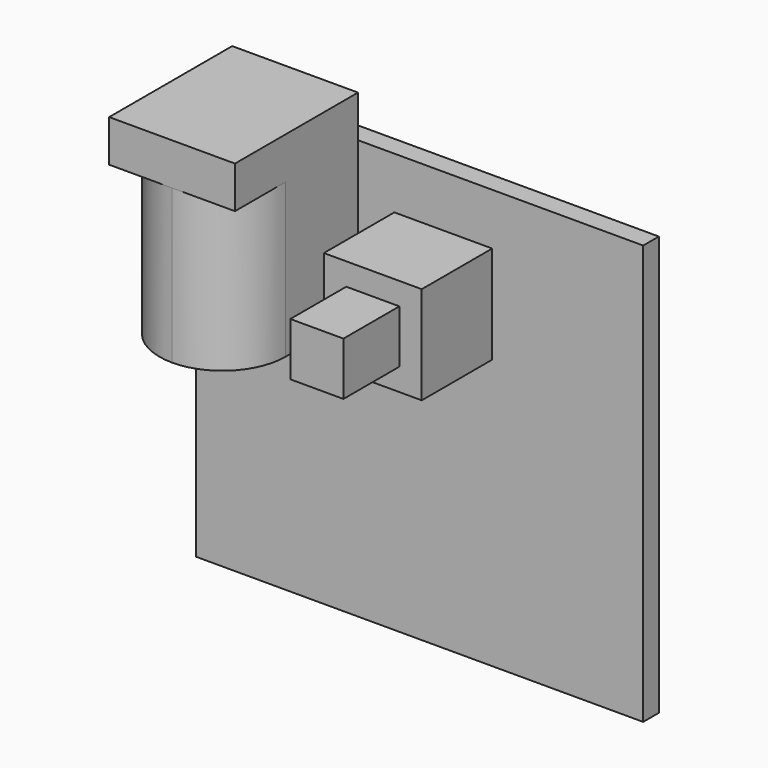
from build123d import *

# Parameters (mm, degrees)
F0_W      = 32
F0_H      = 30
F1_DEPTH  = 1.4
F2_W      = 9
F2_H      = 11
F3_DEPTH  = 11
F4_R      = 4.49999
F6_W      = 7
F6_H      = 7
F7_DEPTH  = 6.3
F8_W      = 3.8
F8_H      = 3.8
F9_DEPTH  = 5
F5_W      = 9
F5_H      = 11
F10_DEPTH = 3


# Not quite as in the source:
# - a fillet or chamfer is up to 0.001 mm smaller than in the source, because OpenCascade refuses the exact size


with BuildPart() as f1:
    # F0 (on Front) → F1 (new body)
    with BuildSketch(Plane.XZ):
        Rectangle(F0_W, F0_H)
    extrude(amount=F1_DEPTH)

    # F2 (on face) → F3 (join)
    with BuildSketch(Plane.XZ.offset(1.4)):
        with Locations((-8.9, 9.5)):
            Rectangle(F2_W, F2_H)
    extrude(amount=F3_DEPTH)

    # F4 (radius 4.5 in the source; OpenCascade refuses exactly that, so slightly less here)
    f4_edges = [f1.edges().sort_by_distance(p)[0] for p in [
        (-4.4, -12.4, 9.5),
        (-13.4, -12.4, 9.5),
    ]]
    fillet(f4_edges, radius=F4_R)

    # F6 (on face) → F7 (join)
    with BuildSketch(Plane.XZ.offset(1.4)):
        with Locations((1.7, 7.8)):
            Rectangle(F6_W, F6_H)
    extrude(amount=F7_DEPTH)

    # F8 (on face) → F9 (join)
    with BuildSketch(Plane.XZ.offset(7.7)):
        with Locations((1.7, 7.8)):
            Rectangle(F8_W, F8_H)
    extrude(amount=F9_DEPTH)

    # F5 (on face) → F10 (join)
    with BuildSketch(Plane.XY.offset(15)):
        with Locations((-8.9, -6.9)):
            Rectangle(F5_W, F5_H)
    extrude(amount=F10_DEPTH)


solid = f1.part
